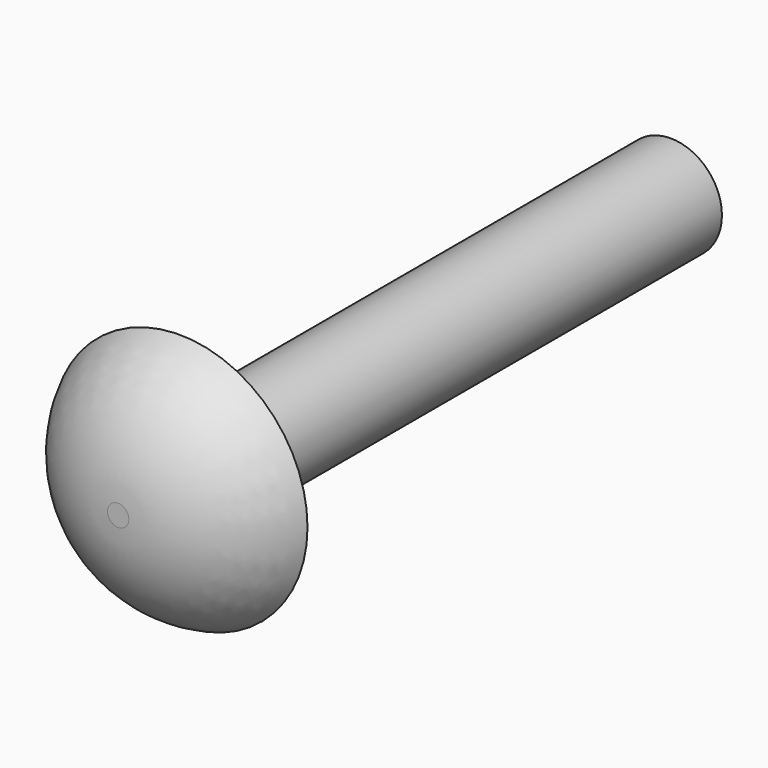
from build123d import *

# Parameters (mm, degrees)
F0_R     = 2
F1_DEPTH = 24
F2_R     = 5
F2_R_2   = 2
F3_DEPTH = 3


# Not quite as in the source:
# - a fillet or chamfer that OpenCascade refuses, or shapes differently, is made with other operations: its cross-section is extruded or revolved along the edge and cut away or added


with BuildPart() as f1:
    # F0 (on Front) → F1 (new body)
    with BuildSketch(Plane.XZ):
        Circle(F0_R)
    extrude(amount=F1_DEPTH)

    # F2 (on face) → F3 (join)
    with BuildSketch(Plane.XZ.offset(24)):
        Circle(F2_R)
        Circle(F2_R_2, mode=Mode.SUBTRACT)
        Circle(F2_R_2)
    extrude(amount=F3_DEPTH)

    # F4: fillet of radius 5 on 1 edges, made by hand

    # F4_s1 → F4_t2 (revolve, cut)
    with BuildSketch(Plane.XY):
        with BuildLine():
            ThreePointArc((5, -24), (3.1560370926, -26.1833001327), (0.417424305, -27))
            Line((0.417424305, -27), (5, -27))
            Line((5, -27), (5, -24))
        make_face()
    revolve(axis=Axis((0, -27, 0), (0, -1, 0)), mode=Mode.SUBTRACT)


solid = f1.part
